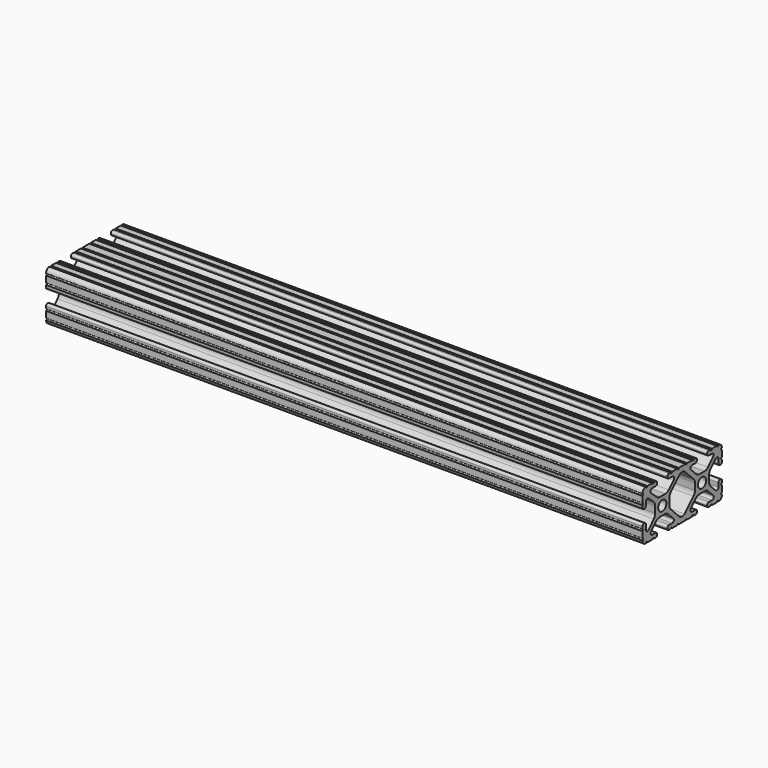
from build123d import *

# Parameters (mm, degrees)
F0_R     = 2.6035
F1_DEPTH = 304.8


# Not quite as in the source:
# - ends of sketch curves that miss each other by under 0.0002 mm in the source are joined


with BuildPart() as f1:
    # F0 (on Right) → F1 (new body)
    with BuildSketch(Plane.YZ):
        with BuildLine():
            ThreePointArc((-16.9874438, -12.7), (-16.2457285259, -12.3927714741), (-15.9385, -11.6510562))
            Line((-15.9385, -11.6510562), (-15.9385, -11.53922))
            ThreePointArc((-15.9385, -11.53922), (-16.2457508444, -10.7974508444), (-16.98752, -10.4902))
            Line((-16.98752, -10.4902), (-19.1163956, -10.4902))
            ThreePointArc((-19.1163956, -10.4902), (-20.0525114102, -9.8690964292), (-19.8440900701, -8.7651747831))
            Line((-19.8440900701, -8.7651747831), (-16.6189914, -5.4551072))
            ThreePointArc((-16.6189914, -5.4551072), (-15.5789897668, -4.7454419004), (-14.3449294, -4.4958))
            Line((-14.3449294, -4.4958), (-11.0833154, -4.4958))
            ThreePointArc((-11.0833154, -4.4958), (-9.8543292721, -4.7433065162), (-8.8169539001, -5.4472374189))
            Line((-8.8169539001, -5.4472374189), (-5.5641494, -8.7626444))
            ThreePointArc((-5.5641494, -8.7626444), (-5.3525969595, -9.8674738324), (-6.2893956, -10.4902))
            Line((-6.2893956, -10.4902), (-8.41248, -10.4902))
            ThreePointArc((-8.41248, -10.4902), (-9.1542491556, -10.7974508444), (-9.4615, -11.53922))
            Line((-9.4615, -11.53922), (-9.4615, -11.6510562))
            ThreePointArc((-9.4615, -11.6510562), (-9.1542714741, -12.3927714741), (-8.4125562, -12.7))
            Line((-8.4125562, -12.7), (-7.382891, -12.7))
            ThreePointArc((-7.382891, -12.7), (-6.874891, -12.192), (-6.366891, -12.7))
            Line((-6.366891, -12.7), (-3.1495746, -12.7))
            ThreePointArc((-3.1495746, -12.7), (-2.6415746, -12.192), (-2.1335746, -12.7))
            Line((-2.1335746, -12.7), (2.1335746, -12.7))
            ThreePointArc((2.1335746, -12.7), (2.6415746, -12.192), (3.1495746, -12.7))
            Line((3.1495746, -12.7), (6.366891, -12.7))
            ThreePointArc((6.366891, -12.7), (6.874891, -12.192), (7.382891, -12.7))
            Line((7.382891, -12.7), (8.4125562, -12.7))
            ThreePointArc((8.4125562, -12.7), (9.1542714741, -12.3927714741), (9.4615, -11.6510562))
            Line((9.4615, -11.6510562), (9.4615, -11.53922))
            ThreePointArc((9.4615, -11.53922), (9.1542491556, -10.7974508444), (8.41248, -10.4902))
            Line((8.41248, -10.4902), (6.2836298, -10.4902))
            ThreePointArc((6.2836298, -10.4902), (5.2972886506, -9.8296334218), (5.5325852439, -8.6660817124))
            Line((5.5325852439, -8.6660817124), (8.80999, -5.4162706))
            ThreePointArc((8.80999, -5.4162706), (9.8367260483, -4.7349218875), (11.0455456, -4.4958))
            Line((11.0455456, -4.4958), (14.3544544, -4.4958))
            ThreePointArc((14.3544544, -4.4958), (15.5632739517, -4.7349218875), (16.5900114796, -5.4162691078))
            Line((16.5900114796, -5.4162691078), (19.8674228, -8.6660736))
            ThreePointArc((19.8674228, -8.6660736), (20.1027113494, -9.8296334218), (19.1163702, -10.4902))
            Line((19.1163702, -10.4902), (16.98752, -10.4902))
            ThreePointArc((16.98752, -10.4902), (16.2457508444, -10.7974508444), (15.9385, -11.53922))
            Line((15.9385, -11.53922), (15.9385, -11.6510562))
            ThreePointArc((15.9385, -11.6510562), (16.2457285259, -12.3927714741), (16.9874438, -12.7))
            Line((16.9874438, -12.7), (18.017109, -12.7))
            ThreePointArc((18.017109, -12.7), (18.525109, -12.192), (19.033109, -12.7))
            Line((19.033109, -12.7), (22.2504, -12.7))
            ThreePointArc((22.2504, -12.7), (22.7583238, -12.1920000057), (23.2663999771, -12.6998476))
            ThreePointArc((23.2663999771, -12.6998476), (24.7825225161, -12.0825225161), (25.3998469825, -10.5664000074))
            ThreePointArc((25.3998469825, -10.5664000074), (24.8920000057, -10.0583238), (25.4, -9.5504))
            Line((25.4, -9.5504), (25.4, -6.3330836))
            ThreePointArc((25.4, -6.3330836), (24.892, -5.8250836), (25.4, -5.3170836))
            Line((25.4, -5.3170836), (25.4, -4.2375074))
            ThreePointArc((25.4, -4.2375074), (25.1073975065, -3.531091972), (24.4009672, -3.2385000003))
            Line((24.4009672, -3.2385000003), (24.23922, -3.2385))
            ThreePointArc((24.23922, -3.2385), (23.4974508444, -3.5457508444), (23.1902, -4.28752))
            Line((23.1902, -4.28752), (23.1902, -6.3347346))
            ThreePointArc((23.1902, -6.3347346), (22.5560286846, -7.2860087813), (21.4340137307, -7.0665132954))
            Line((21.4340137307, -7.0665132954), (18.1479444, -3.8081458))
            ThreePointArc((18.1479444, -3.8081458), (17.4527561757, -2.7748312198), (17.2085, -1.5536164))
            Line((17.2085, -1.5536164), (17.2085, 1.6951706))
            ThreePointArc((17.2085, 1.6951706), (17.4507360791, 2.9115261337), (18.1404815965, 3.9422783948))
            Line((18.1404815965, 3.9422783948), (21.4315802, 7.2273922))
            ThreePointArc((21.4315802, 7.2273922), (22.5544531966, 7.4499349354), (23.1902, 6.4980058))
            Line((23.1902, 6.4980058), (23.1902, 4.28752))
            ThreePointArc((23.1902, 4.28752), (23.4974508444, 3.5457508444), (24.23922, 3.2385))
            Line((24.23922, 3.2385), (24.35098, 3.2385))
            ThreePointArc((24.35098, 3.2385), (25.0927491556, 3.5457508444), (25.4, 4.28752))
            Line((25.4, 4.28752), (25.4, 5.3171344))
            ThreePointArc((25.4, 5.3171344), (24.892, 5.8251344), (25.4, 6.3331344))
            Line((25.4, 6.3331344), (25.4, 9.5504))
            ThreePointArc((25.4, 9.5504), (24.8920000057, 10.0583238), (25.3998476, 10.5663999771))
            ThreePointArc((25.3998476, 10.5663999771), (24.7825225161, 12.0825225161), (23.2664000074, 12.6998469825))
            ThreePointArc((23.2664000074, 12.6998469825), (22.7583238, 12.1920000057), (22.2504, 12.7))
            Line((22.2504, 12.7), (19.0330836, 12.7))
            ThreePointArc((19.0330836, 12.7), (18.5250836, 12.192), (18.0170836, 12.7))
            Line((18.0170836, 12.7), (16.9874692, 12.7))
            ThreePointArc((16.9874692, 12.7), (16.2457000444, 12.3927491556), (15.9384492, 11.65098))
            Line((15.9384492, 11.65098), (15.9384492, 11.53922))
            ThreePointArc((15.9384492, 11.53922), (16.2457000444, 10.7974508444), (16.9874692, 10.4902))
            Line((16.9874692, 10.4902), (19.1163702, 10.4902))
            ThreePointArc((19.1163702, 10.4902), (20.0552104105, 9.8625748951), (19.8341299801, 8.7551194078))
            Line((19.8341299801, 8.7551194078), (16.4966142, 5.4236874))
            ThreePointArc((16.4966142, 5.4236874), (15.4672750099, 4.7369294977), (14.253591, 4.4958))
            Line((14.253591, 4.4958), (11.146409, 4.4958))
            ThreePointArc((11.146409, 4.4958), (9.9327249901, 4.7369294977), (8.9033905965, 5.4236922052))
            Line((8.9033905965, 5.4236922052), (5.5658766, 8.755126))
            ThreePointArc((5.5658766, 8.755126), (5.3447895895, 9.8625748951), (6.2836298, 10.4902))
            Line((6.2836298, 10.4902), (8.4125308, 10.4902))
            ThreePointArc((8.4125308, 10.4902), (9.1542999556, 10.7974508444), (9.4615508, 11.53922))
            Line((9.4615508, 11.53922), (9.4615508, 11.65098))
            ThreePointArc((9.4615508, 11.65098), (9.1542999556, 12.3927491556), (8.4125308, 12.7))
            Line((8.4125308, 12.7), (7.3828656, 12.7))
            ThreePointArc((7.3828656, 12.7), (6.8748656, 12.192), (6.3668656, 12.7))
            Line((6.3668656, 12.7), (3.1496, 12.7))
            ThreePointArc((3.1496, 12.7), (2.6416, 12.192), (2.1336, 12.7))
            Line((2.1336, 12.7), (-2.1336, 12.7))
            ThreePointArc((-2.1336, 12.7), (-2.6416, 12.192), (-3.1496, 12.7))
            Line((-3.1496, 12.7), (-6.3669164, 12.7))
            ThreePointArc((-6.3669164, 12.7), (-6.8749164, 12.192), (-7.3829164, 12.7))
            Line((-7.3829164, 12.7), (-8.4125308, 12.7))
            ThreePointArc((-8.4125308, 12.7), (-9.1542999556, 12.3927491556), (-9.4615508, 11.65098))
            Line((-9.4615508, 11.65098), (-9.4615508, 11.53922))
            ThreePointArc((-9.4615508, 11.53922), (-9.1542999556, 10.7974508444), (-8.4125308, 10.4902))
            Line((-8.4125308, 10.4902), (-6.2893956, 10.4902))
            ThreePointArc((-6.2893956, 10.4902), (-5.2315828864, 9.7830439928), (-5.4806702224, 8.5352487955))
            Line((-5.4806702224, 8.5352487955), (-8.5979254, 5.4236874))
            ThreePointArc((-8.5979254, 5.4236874), (-9.6272645901, 4.7369294977), (-10.8409486, 4.4958))
            Line((-10.8409486, 4.4958), (-14.1025626, 4.4958))
            ThreePointArc((-14.1025626, 4.4958), (-15.2159322292, 4.6974125263), (-16.187903897, 5.276645311))
            Line((-16.187903897, 5.276645311), (-19.8682356, 8.4822538))
            ThreePointArc((-19.8682356, 8.4822538), (-20.1884581676, 9.746870327), (-19.1163956, 10.4902))
            Line((-19.1163956, 10.4902), (-16.9874692, 10.4902))
            ThreePointArc((-16.9874692, 10.4902), (-16.2457000444, 10.7974508444), (-15.9384492, 11.53922))
            Line((-15.9384492, 11.53922), (-15.9384492, 11.65098))
            ThreePointArc((-15.9384492, 11.65098), (-16.2457000444, 12.3927491556), (-16.9874692, 12.7))
            Line((-16.9874692, 12.7), (-18.017109, 12.7))
            ThreePointArc((-18.017109, 12.7), (-18.525109, 12.192), (-19.033109, 12.7))
            Line((-19.033109, 12.7), (-22.2504, 12.7))
            ThreePointArc((-22.2504, 12.7), (-22.7583238, 12.1920000057), (-23.2663999771, 12.6998476))
            ThreePointArc((-23.2663999771, 12.6998476), (-24.7825225161, 12.0825225161), (-25.3998469825, 10.5664000074))
            ThreePointArc((-25.3998469825, 10.5664000074), (-24.8920000057, 10.0583238), (-25.4, 9.5504))
            Line((-25.4, 9.5504), (-25.4, 6.3330836))
            ThreePointArc((-25.4, 6.3330836), (-24.892, 5.8250836), (-25.4, 5.3170836))
            Line((-25.4, 5.3170836), (-25.4, 4.2375074))
            ThreePointArc((-25.4, 4.2375074), (-25.1073810872, 3.5311009523), (-24.4009672, 3.2385))
            Line((-24.4009672, 3.2385), (-24.1892074, 3.2385))
            ThreePointArc((-24.1892074, 3.2385), (-23.4828009523, 3.5311189128), (-23.1902, 4.2375328))
            Line((-23.1902, 4.2375328), (-23.1902, 6.1558678))
            ThreePointArc((-23.1902, 6.1558678), (-22.6223352404, 7.0382408117), (-21.5839937627, 6.8869150285))
            Line((-21.5839937627, 6.8869150285), (-18.29816, 4.0249602))
            ThreePointArc((-18.29816, 4.0249602), (-17.4937263395, 2.946038231), (-17.2085, 1.630807))
            Line((-17.2085, 1.630807), (-17.2085, -1.630807))
            ThreePointArc((-17.2085, -1.630807), (-17.4423469966, -2.8267350959), (-18.109441109, -3.8464967708))
            Line((-18.109441109, -3.8464967708), (-21.5263476, -7.353427))
            ThreePointArc((-21.5263476, -7.353427), (-22.5858996958, -7.5749370688), (-23.1902, -6.6768726))
            Line((-23.1902, -6.6768726), (-23.1902, -4.2375074))
            ThreePointArc((-23.1902, -4.2375074), (-23.4828024935, -3.531091972), (-24.1892328, -3.2385000003))
            Line((-24.1892328, -3.2385000003), (-24.4009672, -3.2385))
            ThreePointArc((-24.4009672, -3.2385), (-25.1073900675, -3.5311099325), (-25.4, -4.2375328))
            Line((-25.4, -4.2375328), (-25.4, -5.3170836))
            ThreePointArc((-25.4, -5.3170836), (-24.8919492, -5.8251344), (-25.4, -6.3331852))
            Line((-25.4, -6.3331852), (-25.4, -9.5504))
            ThreePointArc((-25.4, -9.5504), (-24.8920000057, -10.0583238), (-25.3998476, -10.5663999771))
            ThreePointArc((-25.3998476, -10.5663999771), (-24.7825225161, -12.0825225161), (-23.2664000074, -12.6998469825))
            ThreePointArc((-23.2664000074, -12.6998469825), (-22.7583238, -12.1920000057), (-22.2504, -12.7))
            Line((-22.2504, -12.7), (-19.033109, -12.7))
            ThreePointArc((-19.033109, -12.7), (-18.525109, -12.192), (-18.017109, -12.7))
            Line((-18.017109, -12.7), (-16.9874438, -12.7))
        make_face()
        with Locations((-12.7, 0)):
            Circle(F0_R, mode=Mode.SUBTRACT)
        with BuildLine():
            Line((1.5457424, 9.5727774), (7.2595232, 3.8694106))
            ThreePointArc((7.2595232, 3.8694106), (7.9492639209, 2.8386535337), (8.1915, 1.622298))
            Line((8.1915, 1.622298), (8.1915, -1.622298))
            ThreePointArc((8.1915, -1.622298), (7.9472438243, -2.8435128198), (7.2520570796, -3.8768288922))
            Line((7.2520570796, -3.8768288922), (1.5040356, -9.5764604))
            ThreePointArc((1.5040356, -9.5764604), (0.9947690665, -9.9143972036), (0.3951986, -10.033))
            Line((0.3951986, -10.033), (-0.5514594, -10.033))
            ThreePointArc((-0.5514594, -10.033), (-1.1610302602, -9.9102393956), (-1.6755651956, -9.5610967315))
            Line((-1.6755651956, -9.5610967315), (-7.2828658, -3.8458648))
            ThreePointArc((-7.2828658, -3.8458648), (-7.9555749193, -2.8233240692), (-8.1915, -1.622298))
            Line((-8.1915, -1.622298), (-8.1915, 1.622298))
            ThreePointArc((-8.1915, 1.622298), (-7.9492639209, 2.8386535337), (-7.2595184035, 3.8694057948))
            Line((-7.2595184035, 3.8694057948), (-1.5457424, 9.5727774))
            ThreePointArc((-1.5457424, 9.5727774), (-1.0352001727, 9.9134036975), (-0.4332224, 10.033))
            Line((-0.4332224, 10.033), (0.4332224, 10.033))
            ThreePointArc((0.4332224, 10.033), (1.0352001727, 9.9134036975), (1.5457424, 9.5727774))
        make_face(mode=Mode.SUBTRACT)
        with Locations((12.7, 0)):
            Circle(F0_R, mode=Mode.SUBTRACT)
    extrude(amount=-F1_DEPTH)


solid = f1.part
